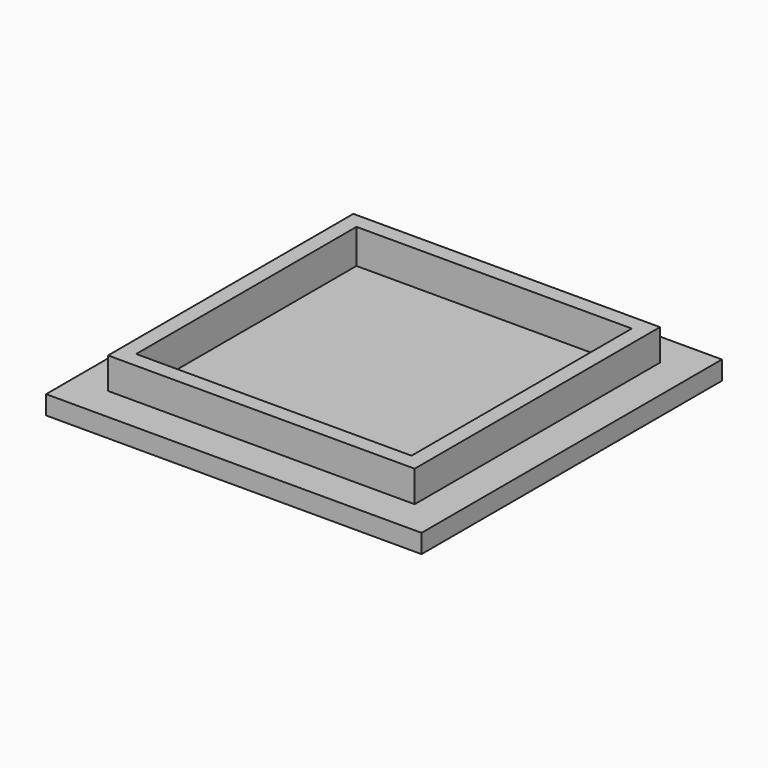
from build123d import *

# Parameters (mm, degrees)
F0_W        = 60
F0_H        = 60
F1_DEPTH    = 3
F2_W        = 49
F2_H        = 49
F3_DEPTH    = 5
F4_T        = 2.5
F4_T3_DEPTH = 54
F4_T5_DEPTH = 54


# Not quite as in the source:
# - a shell that OpenCascade refuses in one call is made with other operations: the cavity is built on its own and cut out


with BuildPart() as f1:
    # F0 (on Top) → F1 (new body)
    with BuildSketch(Plane.XY):
        Rectangle(F0_W, F0_H)
    extrude(amount=F1_DEPTH)

    # F2 (on face) → F3 (join)
    with BuildSketch(Plane.XY.offset(3)):
        Rectangle(F2_W, F2_H)
    extrude(amount=F3_DEPTH)

    # F4: shell of thickness 2.5, made by hand


with BuildPart() as f4_core1:
    # F4_t2: copy of F1
    add(f1.part)

    # the walls: a layer under each face that stays
    f4_faces = [f4_core1.faces().sort_by_distance(p)[0] for p in [
        (0, -30, 1.5),
        (-30, 0, 1.5),
        (30, 0, 1.5),
        (0, 0, 0),
        (-25.7142857143, -25.7142857143, 3),
        (0, 30, 1.5),
        (0, -24.5, 5.5),
        (24.5, 0, 5.5),
        (0, 24.5, 5.5),
        (-24.5, 0, 5.5),
    ]]
    thicken(f4_faces, amount=-F4_T, mode=Mode.SUBTRACT)

    # F4_s4 → F4_t3 (cut)
    with BuildSketch(Plane.YZ.offset(-27)):
        Polygon((-24.525, 3.025), (-24.5, 0.5), (-22, 0.5), (-22, 3), align=None)
        Polygon((24.525, 3.025), (24.5, 0.5), (22, 0.5), (22, 3), align=None)
    extrude(amount=F4_T3_DEPTH, mode=Mode.SUBTRACT)

    # F4_s6 → F4_t5 (cut)
    with BuildSketch(Plane.XZ.offset(-27)):
        Polygon((24.525, 3.025), (24.5, 0.5), (22, 0.5), (22, 3), align=None)
        Polygon((-24.525, 3.025), (-24.5, 0.5), (-22, 0.5), (-22, 3), align=None)
    extrude(amount=F4_T5_DEPTH, mode=Mode.SUBTRACT)


with BuildPart() as f1_1:
    add(f1.part)

    # what is left inside the walls is the cavity
    f4_cavity = [f4_core1.part.solids().sort_by_distance(p)[0] for p in [
        (0, -7.333333, 2.525),
    ]]
    add(f4_cavity, mode=Mode.SUBTRACT)


solid = f1_1.part
